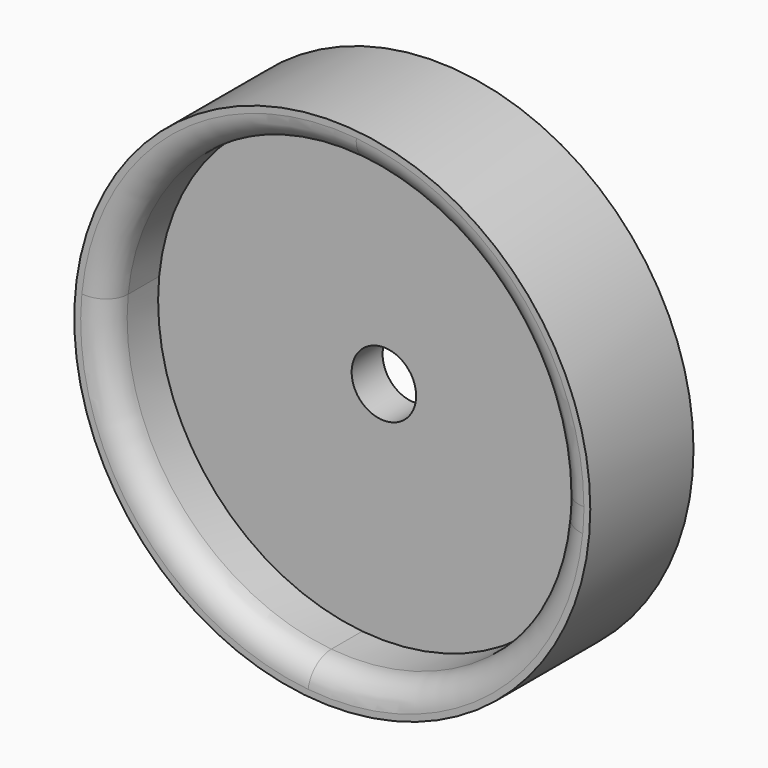
from build123d import *

# Parameters (mm, degrees)
F0_R     = 20
F1_DEPTH = 10
F2_START = 2
F2_DEPTH = 3
F3_R     = 1.99999
F4_D     = 5


# Not quite as in the source:
# - a fillet or chamfer is up to 0.001 mm smaller than in the source, because OpenCascade refuses the exact size


with BuildPart() as f1:
    # F0 (on Front) → F1 (new body)
    with BuildSketch(Plane.XZ):
        Circle(F0_R)
        with BuildLine():
            ThreePointArc((1.6759297538, 17.4195654211), (12.9533542122, 11.766928854), (17.5, 0))
            ThreePointArc((17.5, 0), (17.4798797889, -0.8389294162), (17.4195654211, -1.6759297538))
            ThreePointArc((17.4195654211, -1.6759297538), (11.1324315409, -13.5025541283), (-1.6759297538, -17.4195654211))
            ThreePointArc((-1.6759297538, -17.4195654211), (-13.5025541283, -11.1324315409), (-17.4195654211, 1.6759297538))
            ThreePointArc((-17.4195654211, 1.6759297538), (-11.1324315409, 13.5025541283), (1.6759297538, 17.4195654211))
        make_face(mode=Mode.SUBTRACT)
    extrude(amount=F1_DEPTH)

    # F0 (on Front) → F2 (join)
    with BuildSketch(Plane.XZ.offset(F2_START)):
        with BuildLine():
            Line((0, 0), (1.6759297538, 17.4195654211))
            ThreePointArc((1.6759297538, 17.4195654211), (-11.1324315409, 13.5025541283), (-17.4195654211, 1.6759297538))
            Line((-17.4195654211, 1.6759297538), (0, 0))
        make_face()
        with BuildLine():
            ThreePointArc((-1.6759297538, -17.4195654211), (11.1324315409, -13.5025541283), (17.4195654211, -1.6759297538))
            Line((17.4195654211, -1.6759297538), (0, 0))
            Line((0, 0), (-1.6759297538, -17.4195654211))
        make_face()
        with BuildLine():
            Line((0, 0), (-17.4195654211, 1.6759297538))
            ThreePointArc((-17.4195654211, 1.6759297538), (-13.5025541283, -11.1324315409), (-1.6759297538, -17.4195654211))
            Line((-1.6759297538, -17.4195654211), (0, 0))
        make_face()
        with BuildLine():
            ThreePointArc((17.4195654211, -1.6759297538), (17.4798797889, -0.8389294162), (17.5, 0))
            ThreePointArc((17.5, 0), (12.9533542122, 11.766928854), (1.6759297538, 17.4195654211))
            Line((1.6759297538, 17.4195654211), (0, 0))
            Line((0, 0), (17.4195654211, -1.6759297538))
        make_face()
    extrude(amount=F2_DEPTH)

    # F3 (radius 2 in the source; OpenCascade refuses exactly that, so slightly less here)
    f3_edges = [f1.edges().sort_by_distance(p)[0] for p in [
        (-17.5, -10, 0),
        (-17.5, 0, 0),
    ]]
    fillet(f3_edges, radius=F3_R)

    # F4 (through all)
    with Locations(Plane(origin=(0, 0, 0), x_dir=(1, 0, 0), z_dir=(0, 1, 0))):
        with Locations((0, 0)):
            Hole(F4_D / 2)


solid = f1.part
